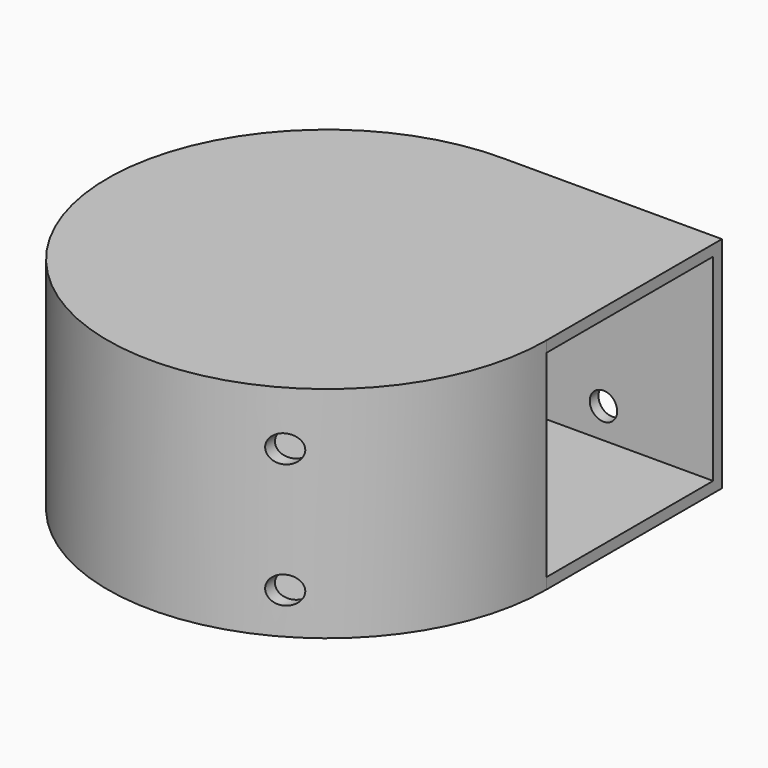
from build123d import *

# Parameters (mm, degrees)
F0_W      = 50.8
F0_H      = 50.8
F1_DEPTH  = 25.4
F1_FACE_W = 50.8
F1_FACE_H = 50.8
F3_T      = -2.54
F5_D      = 6.35


# Not quite as in the source:
# - a shell that OpenCascade refuses in one call is made with other operations: the cavity is built on its own and cut out


with BuildPart() as f1:
    # F0 (on Front) → F1 (new body, symmetric)
    with BuildSketch(Plane.XZ):
        Rectangle(F0_W, F0_H)
    extrude(amount=F1_DEPTH, both=True)

    # F1_face (on face) → F2 (revolve)
    with BuildSketch(Plane.XZ.offset(25.4)):
        Rectangle(F1_FACE_W, F1_FACE_H)
    revolve(axis=Axis((-25.4, -25.4, 0), (0, 0, 1)))

    # F3: a shell. OpenCascade refuses it in one call, so the cavity is built on its own and cut out:
    # the body offset inwards by the wall thickness, plus a prism from it out through each open face.
    f3_core = offset(f1.part, amount=F3_T, mode=Mode.PRIVATE)
    f3_exits = [f3_core.faces().sort_by_distance(p)[0] for p in [
        (22.86, -1.27, 0),
    ]]
    add(f3_core, mode=Mode.SUBTRACT)
    extrude(f3_exits, amount=-F3_T, mode=Mode.SUBTRACT)

    # F5 (through all)
    with Locations(Plane(origin=(0, 25.4, 0), x_dir=(-1, 0, 0), z_dir=(0, 1, 0))):
        with Locations((0, 12.914407067), (0, -15.8760398626)):
            Hole(F5_D / 2)


solid = f1.part
